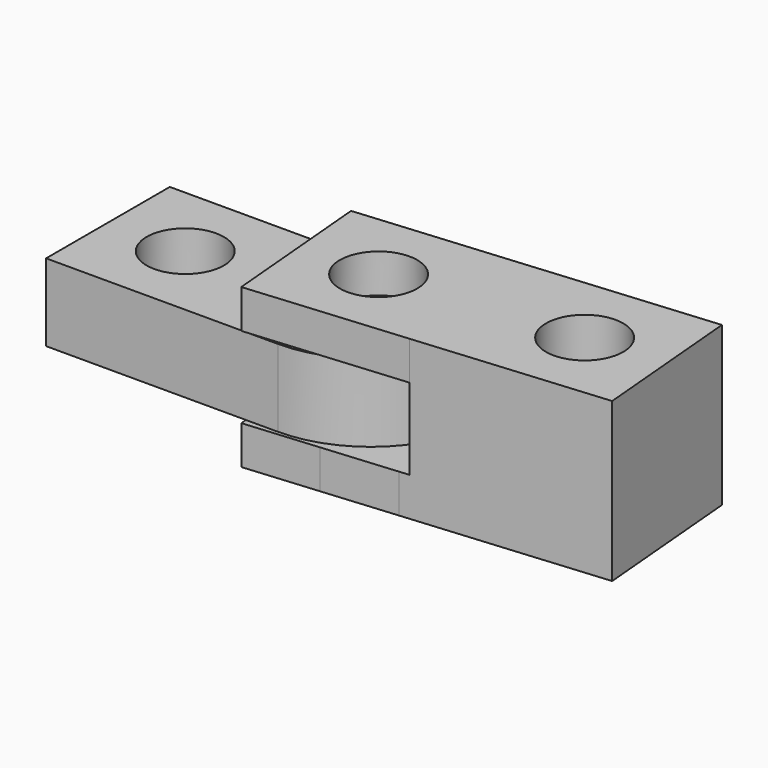
from build123d import *

# Parameters (mm, degrees)
F0_W     = 90
F0_H     = 40
F0_R     = 10
F1_DEPTH = 20
F2_R     = 10
F3_DEPTH = 10
F5_DEPTH = 30.001
F6_R     = 10
F7_DEPTH = 21
F8_R     = 10
F9_DEPTH = 10


with BuildPart() as f1:
    # F0 (on Top) → F1 (new body)
    with BuildSketch(Plane.XY):
        with Locations((25, 0)):
            Rectangle(F0_W, F0_H)
        Circle(F0_R, mode=Mode.SUBTRACT)
        with Locations((50, 0)):
            Circle(F0_R, mode=Mode.SUBTRACT)
    extrude(amount=F1_DEPTH)

    # F4 (on face) → F5 (cut, through all)
    with BuildSketch(Plane.XY.offset(20)):
        with BuildLine():
            Line((70, -20), (70, 10))
            ThreePointArc((70, 10), (61.2132034356, -11.2132034356), (40, -20))
            Line((40, -20), (70, -20))
        make_face()
    extrude(amount=-F5_DEPTH, mode=Mode.SUBTRACT)


with BuildPart() as f3:
    # F2 (on face) → F3 (new body)
    with BuildSketch(Plane(origin=(0, 0, 0), x_dir=(1, 0, 0), z_dir=(0, 0, -1))):
        Polygon((50.8732188582, 20), (31.8192208931, 21.6670088168), (31.6733765197, 20), align=None)
        Polygon((70, 18.3266234803), (50.8732188582, 20), (31.6733765197, 20), (28.3329911832, -18.1807791069), (49.1267811418, -20), (70, -20), align=None)
        with Locations((50, 0)):
            Circle(F2_R, mode=Mode.SUBTRACT)
        Polygon((121.4767437214, 13.8229919695), (70, 18.3266234803), (70, -20), (49.1267811418, -20), (117.9905140115, -26.0247959542), align=None)
        with Locations((99.8097349046, -4.3577871374)):
            Circle(F2_R, mode=Mode.SUBTRACT)
    extrude(amount=F3_DEPTH)

    # F6 (on face) → F7 (join)
    with BuildSketch(Plane.XY):
        Polygon((70, 21.8261700214), (70, 20), (70, 10), (72.4594332734, -18.1114509502), (121.4767437214, -13.8229919695), (117.9905140115, 26.0247959542), align=None)
        with Locations((99.8097349046, 4.3577871374)):
            Circle(F6_R, mode=Mode.SUBTRACT)
    extrude(amount=F7_DEPTH)

    # F8 (on face) → F9 (join)
    with BuildSketch(Plane.XY.offset(21)):
        Polygon((70, 10), (72.4594332734, -18.1114509502), (121.4767437214, -13.8229919695), (117.9905140115, 26.0247959542), (70, 21.8261700214), align=None)
        with Locations((99.8097349046, 4.3577871374)):
            Circle(F8_R, mode=Mode.SUBTRACT)
        Polygon((28.3329911832, 18.1807791069), (31.8192208931, -21.6670088168), (72.4594332734, -18.1114509502), (70, 10), (70, 21.8261700214), align=None)
        with Locations((50, 0)):
            Circle(F8_R, mode=Mode.SUBTRACT)
    extrude(amount=F9_DEPTH)


solid = Compound([f1.part, f3.part])
